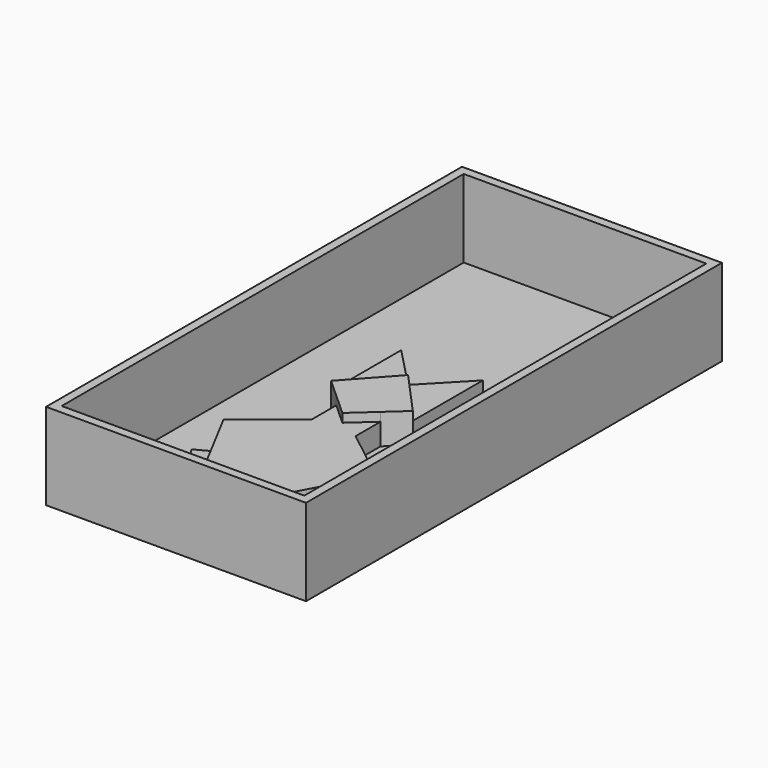
from build123d import *

# Parameters (mm, degrees)
F0_W      = 76.2
F0_H      = 152.4
F1_DEPTH  = 25.4
F2_T      = -2.54
F4_DEPTH  = 6.35
F6_DEPTH  = 8.89
F8_DEPTH  = 6.35
F10_DEPTH = 3.81


# Not quite as in the source:
# - a pattern or mirror of a feature is missing from the dataset's text; its kind, count and spacing are read off the source's solid


with BuildPart() as f1:
    # F0 (on Top) → F1 (new body)
    with BuildSketch(Plane.XY):
        with Locations((0, 76.2)):
            Rectangle(F0_W, F0_H)
    extrude(amount=F1_DEPTH)

    # F2
    f2_openings = [f1.faces().sort_by_distance(p)[0] for p in [
        (0, 76.2, 25.4),
    ]]
    offset(amount=F2_T, openings=f2_openings)

    # F3 (on face) → F4 (join)
    with BuildSketch(Plane.XY.offset(2.54)):
        Polygon((-6.4988862723, 57.677667588), (-22.2837403417, 45.2752783895), (-3.4451077227, 9.7248451784), (-7.3955161497, 2.54), (7.3955161497, 2.54), (3.4451077227, 9.7248451784), (22.2837403417, 45.2752783895), (6.4988862723, 57.677667588), (6.4988862723, 66.8228566647), (0, 60.9430685656), (-6.4988862723, 66.8228566647), align=None)
    extrude(amount=F4_DEPTH)

    # F5 (on face) → F6 (join)
    with BuildSketch(Plane.XY.offset(2.54)):
        Polygon((-6.4988862723, 66.8228566647), (0, 60.9430685656), (6.4988862723, 66.8228566647), (11.9773805831, 71.7794575804), (0, 85.0179677), (-11.9773805831, 71.7794575804), align=None)
    extrude(amount=F6_DEPTH)

    # F7 (on face) → F8 (join)
    with BuildSketch(Plane.XY.offset(2.54)):
        Polygon((11.9773805831, 97.4589511752), (0, 85.0179677), (11.9773805831, 71.7794575804), align=None)
        Polygon((-11.9773805831, 97.4589511752), (-11.9773805831, 71.7794575804), (0, 85.0179677), align=None)
    extrude(amount=F8_DEPTH)

    # F9 (on face) → F10 (join)
    with BuildSketch(Plane.XY.offset(2.54)):
        Polygon((-3.4451077227, 9.7248451784), (-17.0620636054, 35.4214384736), (-21.7691510916, 32.9270921648), (-8.3730621263, 10.7017857954), (-11.2379649654, 6.5747052431), (-9.2242012438, 2.7745264226), (-7.3955161497, 2.54), align=None)
    f10 = extrude(amount=F10_DEPTH)

    # F10_copies: F10 across plane
    add(f10.mirror(Plane(origin=(0, 0, 0), x_dir=(0, 0, 1), z_dir=(1, 0, 0))))


solid = f1.part
